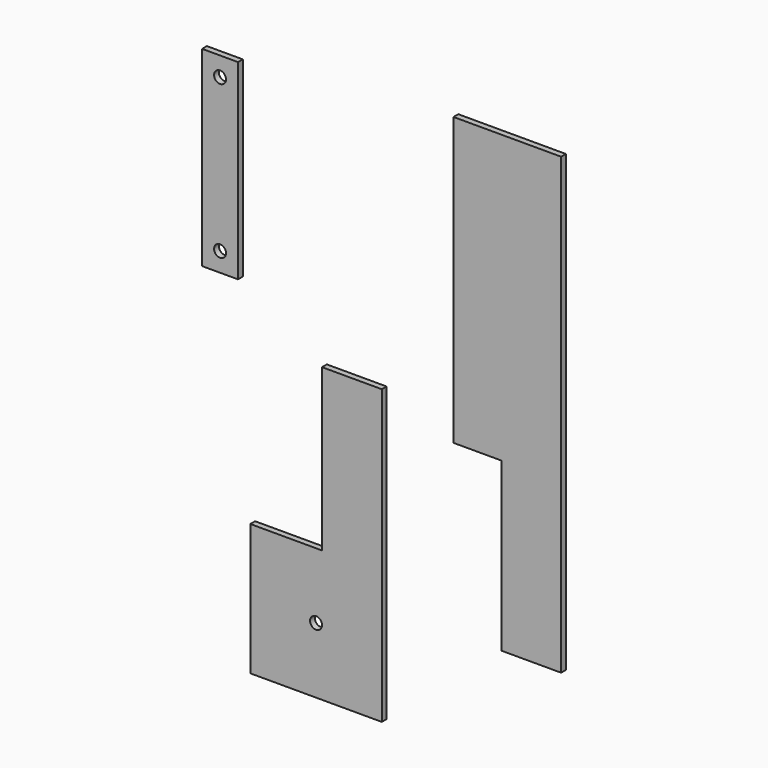
from build123d import *

# Parameters (mm, degrees)
F1_DEPTH  = 3.175
F3_DEPTH  = 3.175
F4_DEPTH  = 31.75
F5_DEPTH  = 12.7
F6_R      = 3.175
F7_DEPTH  = 25.4
F8_W      = 19.05
F8_H      = 101.6
F9_DEPTH  = 3.175
F10_R     = 3.175
F11_DEPTH = 25.4


with BuildPart() as f1:
    # F0 (on Front) → F1 (new body)
    with BuildSketch(Plane.XZ):
        Polygon((57.15, 152.4), (0, 152.4), (0, 0), (25.4, 0), (25.4, -88.9), (57.15, -88.9), (57.15, 0), align=None)
    extrude(amount=F1_DEPTH)


with BuildPart() as f3:
    # F2 (on Front) → F3 (new body)
    with BuildSketch(Plane.XZ):
        Polygon((-38.1, 0), (-69.85, 0), (-69.85, -73.025), (-107.95, -73.025), (-107.95, -111.125), (-69.85, -111.125), (-38.1, -111.125), (-38.1, -73.025), align=None)
    extrude(amount=F3_DEPTH)

    # F4 (add): a face of the model
    f4_faces = [f3.faces().sort_by_distance(p)[0] for p in [
        (-73.025, -1.5875, -111.125),
    ]]
    extrude(f4_faces, amount=F4_DEPTH)

    # F5 (add): a face of the model
    f5_faces = [f3.faces().sort_by_distance(p)[0] for p in [
        (-53.975, -1.5875, 0),
    ]]
    extrude(f5_faces, amount=F5_DEPTH)

    # F6 (on face) → F7 (cut)
    with BuildSketch(Plane.XZ.offset(3.175)):
        with Locations((-73.025, -107.95)):
            Circle(F6_R)
    extrude(amount=-F7_DEPTH, mode=Mode.SUBTRACT)


with BuildPart() as f9:
    # F8 (on Front) → F9 (new body)
    with BuildSketch(Plane.XZ):
        with Locations((-124.0121312439, 90.0274350342)):
            Rectangle(F8_W, F8_H)
    extrude(amount=F9_DEPTH)

    # F10 (on face) → F11 (cut)
    with BuildSketch(Plane.XZ.offset(3.175)):
        with Locations((-124.0121312439, 130.6674350342)):
            Circle(F10_R)
        with Locations((-124.0121312439, 49.3874350342)):
            Circle(F10_R)
    extrude(amount=-F11_DEPTH, mode=Mode.SUBTRACT)


solid = Compound([f1.part, f3.part, f9.part])
